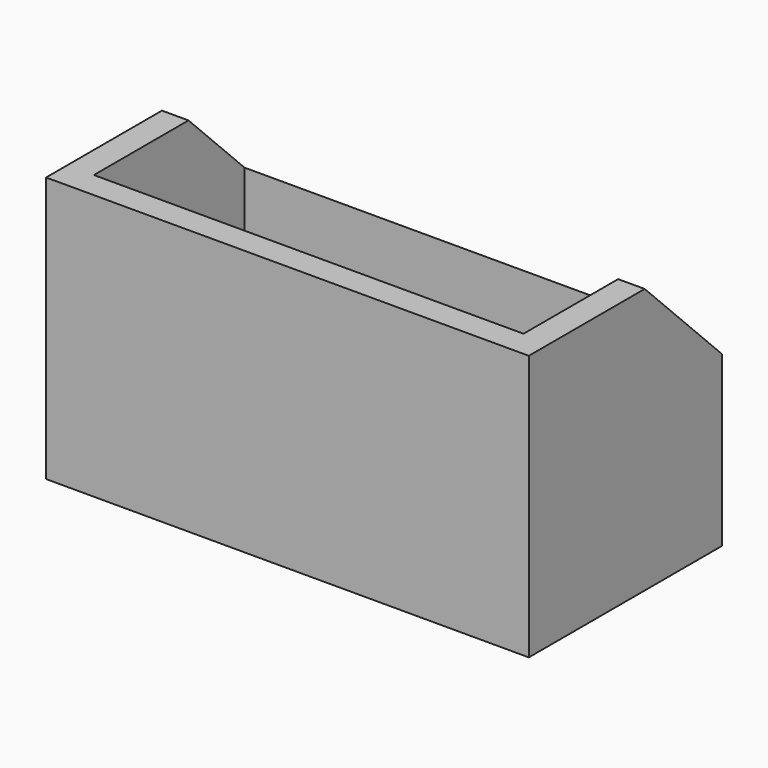
from build123d import *

# Parameters (mm, degrees)
F0_W        = 100
F0_H        = 55
F1_DEPTH    = 50
F2_T        = -5.5
F3_T1_DEPTH = 202.8673195186


# Not quite as in the source:
# - a fillet or chamfer that OpenCascade refuses, or shapes differently, is made with other operations: its cross-section is extruded or revolved along the edge and cut away or added


with BuildPart() as f1:
    # F0 (on Front) → F1 (new body)
    with BuildSketch(Plane.XZ):
        Rectangle(F0_W, F0_H)
    extrude(amount=F1_DEPTH)

    # F2
    f2_openings = [f1.faces().sort_by_distance(p)[0] for p in [
        (0, -25, 27.5),
    ]]
    offset(amount=F2_T, openings=f2_openings)

    # F3: chamfer of 20 on 1 edges, made by hand

    # F3_s2 → F3_t1 (cut)
    with BuildSketch(Plane.YZ.offset(-101.4336597593)):
        Polygon((0, 7.5), (-20, 27.5), (0, 27.5), align=None)
    extrude(amount=F3_T1_DEPTH, mode=Mode.SUBTRACT)


solid = f1.part
